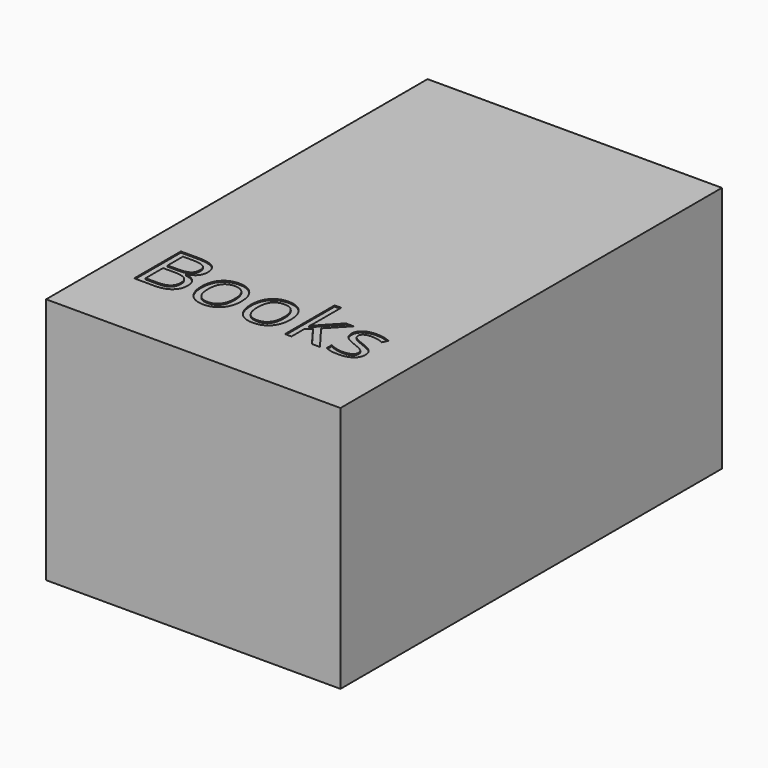
from build123d import *

# Parameters (mm, degrees)
F0_W         = 250
F0_H         = 405
F1_DEPTH     = 210
F2_TEXT_SIZE = 69.4444444444
F3_DEPTH     = 1


# Not quite as in the source:
# - Text() gives the source's letters only with a copy of the font that has no kerning and outlines rounded to 1/6400 em; it was checked with that copy


with BuildPart() as f1:
    # F0 (on Top) → F1 (new body)
    with BuildSketch(Plane.XY):
        Rectangle(F0_W, F0_H)
    extrude(amount=F1_DEPTH)

    # F2 (on face) → F3 (cut)
    with BuildSketch(Plane.XY.offset(210)):
        with Locations((-105, -142.5)):
            Text('Books', F2_TEXT_SIZE, font='Open Sans', text_align=(TextAlign.LEFT, TextAlign.BOTTOM))
    extrude(amount=-F3_DEPTH, mode=Mode.SUBTRACT)


solid = f1.part
